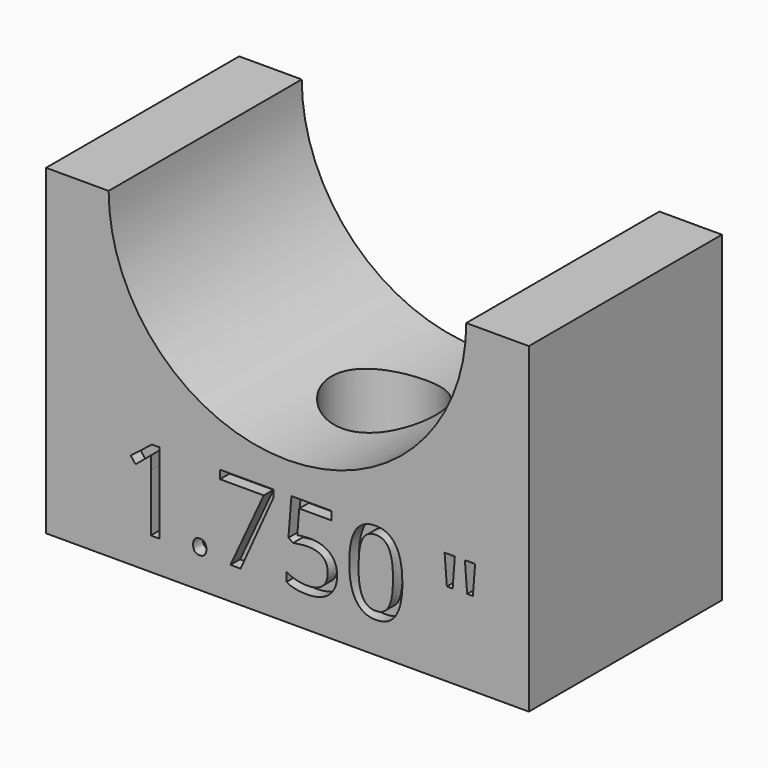
from build123d import *

# Parameters (mm, degrees)
F1_DEPTH       = 30
F3_D           = 9
F3_START       = 2.2250001
F3_CBORE_D     = 13
F3_CBORE_DEPTH = 9
F4_TEXT_SIZE   = 14.0030145379
F5_DEPTH       = 1.5


# Not quite as in the source:
# - Text() gives the source's letters only with a copy of the font that has no kerning and outlines rounded to 1/6400 em; it was checked with that copy


with BuildPart() as f1:
    # F0 (on Front) → F1 (new body)
    with BuildSketch(Plane.XZ):
        with BuildLine():
            Line((-30, -20), (30, -20))
            Line((30, -20), (30, 20))
            Line((30, 20), (22.225, 20))
            ThreePointArc((22.225, 20), (0, -2.225), (-22.225, 20))
            Line((-22.225, 20), (-30, 20))
            Line((-30, 20), (-30, -20))
        make_face()
    extrude(amount=F1_DEPTH)

    # F3 (through all)
    # its depths count from where the whole tool has entered the part; down to there all is cleared
    with Locations(Plane.XY.offset(-F3_START)):
        with Locations((0, -15)):
            CounterBoreHole(F3_D / 2, F3_CBORE_D / 2, F3_CBORE_DEPTH)

    # F4 (on face) → F5 (cut)
    with BuildSketch(Plane.XZ.offset(30)):
        with Locations((-20.7662621453, -16)):
            Text('1.750 "', F4_TEXT_SIZE, font='Open Sans', text_align=(TextAlign.LEFT, TextAlign.BOTTOM))
    extrude(amount=-F5_DEPTH, mode=Mode.SUBTRACT)


solid = f1.part
